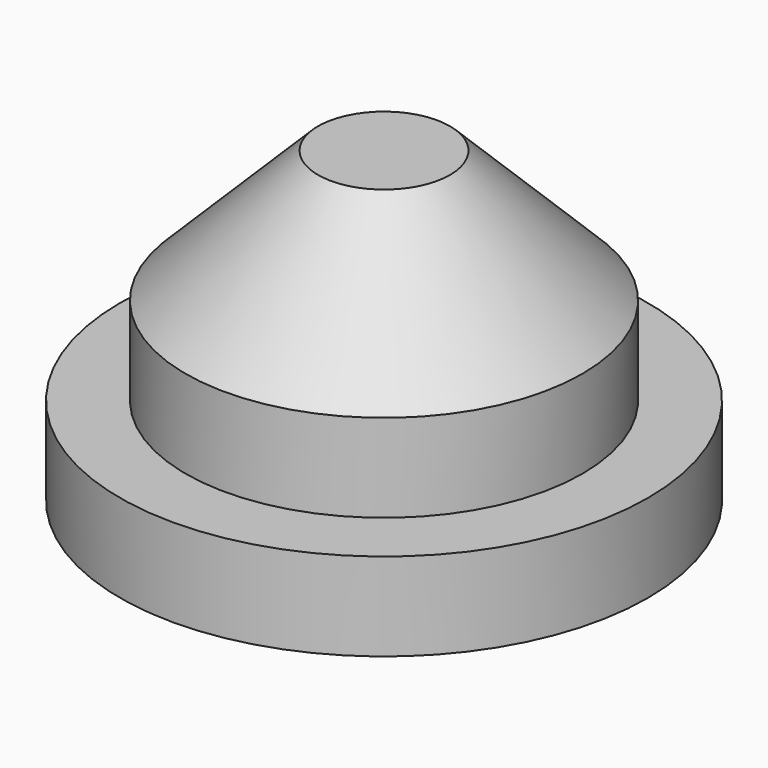
from build123d import *

# Parameters (mm, degrees)
F0_R     = 12.7
F1_DEPTH = 7.62
F3_DEPTH = 5.08
F7_R     = 15.24
F8_DEPTH = 5.08


# Not quite as in the source:
# - a fillet or chamfer that OpenCascade refuses, or shapes differently, is made with other operations: its cross-section is extruded or revolved along the edge and cut away or added
# - the program builds the solid bodies; features that only make, move or delete a surface that nothing else refers to are left out


with BuildPart() as f1:
    # F0 (on Top) → F1 (new body)
    with BuildSketch(Plane.XY):
        Circle(F0_R)
    extrude(amount=F1_DEPTH)

    # F2: chamfer of 8.89 x 8.8590220811 on 1 edges, made by hand

    # F2_s1 → F2_t2 (revolve, cut)
    with BuildSketch(Plane.XZ):
        Polygon((12.7, -1.2390220811), (3.81, 7.62), (12.7, 7.62), align=None)
    revolve(axis=Axis((0, 0, 7.62), (0, 0, 1)), mode=Mode.SUBTRACT)

    # F3 (add): a face of the model
    f3_faces = [f1.faces().sort_by_distance(p)[0] for p in [
        (0, 0, 0),
    ]]
    extrude(f3_faces, amount=F3_DEPTH)

    # F7 (on face) → F8 (join)
    with BuildSketch(Plane(origin=(0, 0, -5.08), x_dir=(1, 0, 0), z_dir=(0, 0, -1))):
        Circle(F7_R)
    extrude(amount=F8_DEPTH)


solid = f1.part
